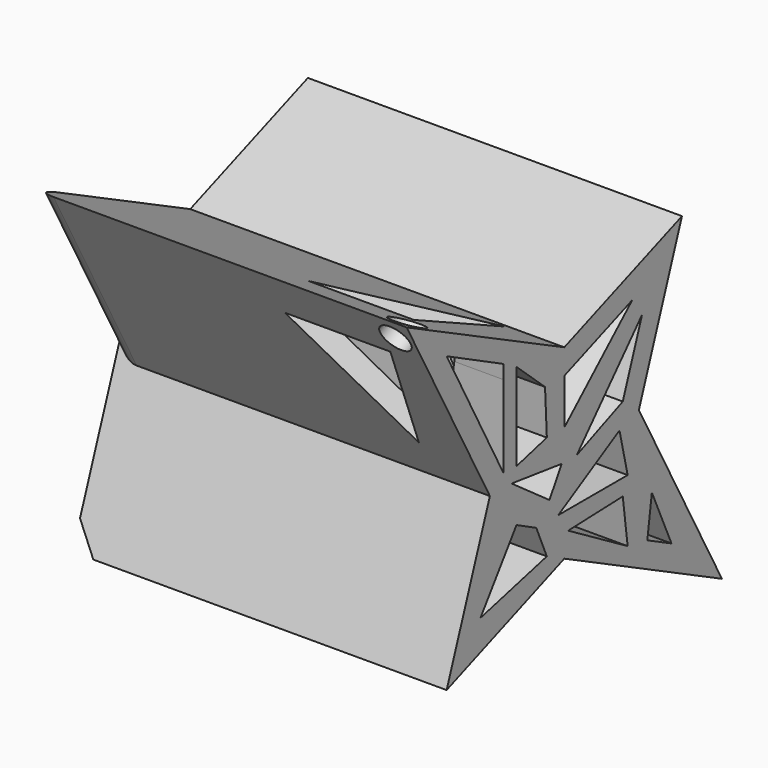
from build123d import *

# Parameters (mm, degrees)
F1_DEPTH    = 22.86
F3_DEPTH    = 22.861
F5_DEPTH    = 21.1407149532
F6_R        = 0.9322227143
F7_DEPTH    = 21.1407149532
F8_R        = 1.27
F9_T4_DEPTH = 16.1477728221


# Not quite as in the source:
# - a fillet or chamfer that OpenCascade refuses, or shapes differently, is made with other operations: its cross-section is extruded or revolved along the edge and cut away or added
# - a feature names something its author has since deleted; it is built from what else it names


with BuildPart() as f1:
    # F0 (on Right) → F1 (new body)
    with BuildSketch(Plane.YZ):
        Polygon((0, 5.6908354163), (-12.0390886441, 11.6551341489), (-5.6838279371, 0), (-8.9875673875, -9.0952031314), (0, -5.6768290866), (12.0390886441, -11.6551341489), (5.6978515349, 0), (8.9875673875, 9.0952031314), align=None)
    extrude(amount=F1_DEPTH)

    # F2 (on face) → F3 (cut, through all)
    with BuildSketch(Plane.YZ.offset(22.86)):
        Polygon((0.2947798819, -4.2920547475), (4.8379492509, -6.9700027277), (4.4653764926, -4.1452315636), align=None)
        Polygon((-0.460864554, -3.1500807424), (4.8379492509, -3.1500807424), (4.2156420195, -0.4934913878), align=None)
        Polygon((-6.4040375873, -6.2635522336), (-1.3339594007, -5.0133955665), (-2.1420896955, -3.1500807424), (-3.6510264616, -2.3839071877), align=None)
        Polygon((-3.6510264616, 0.7806772021), (-1.3339594007, 1.3762915041), (-1.4712439905, 4.1567722153), (-3.6510264616, 6.1231630373), align=None)
        Polygon((-8.9875673875, 8.8637409893), (-4.6268783625, 0.7806772021), (-4.6268783625, 5.8275670744), (-4.6572963607, 6.6916077305), align=None)
        Polygon((0.9543706066, -0.4934913878), (4.4653764926, 0.9595727897), (5.9346228684, 5.0216543911), align=None)
        Polygon((0, 1.3762915041), (5.1912929219, 6.1231630373), (0, 4.1567722153), align=None)
        Polygon((-0.1954076109, -0.4954853684), (-4.0261200629, 0), (-1.1355356546, -2.0616382826), align=None)
        Polygon((8.1868149158, -8.1874002878), (6.6878763027, -4.839763511), (6.3406112604, -7.2706225328), align=None)
    extrude(amount=-F3_DEPTH, mode=Mode.SUBTRACT)

    # F4 (on face) → F5 (cut, through all)
    with BuildSketch(Plane(origin=(0, -4.381188718, -2.3889554726), x_dir=(1, 0, 0), z_dir=(0, -0.8779615957, -0.4787310691))):
        Polygon((20.7448676229, 13.0785638466), (14.3051566556, 13.0785638466), (19.5283554494, 5.3454530425), align=None)
    extrude(amount=-F5_DEPTH, mode=Mode.SUBTRACT)

    # F6 (on face) → F7 (cut, through all)
    with BuildSketch(Plane(origin=(0, -4.381188718, -2.3889554726), x_dir=(1, 0, 0), z_dir=(0, -0.8779615957, -0.4787310691))):
        with Locations((21.6227080673, 14.5550044253)):
            Circle(F6_R)
    extrude(amount=-F7_DEPTH, mode=Mode.SUBTRACT)

    # F8
    f8_edges = [f1.edges().sort_by_distance(p)[0] for p in [
        (0, -8.861458, 5.827567),
    ]]
    fillet(f8_edges, radius=F8_R)

    # F9: chamfer of 1.27 on 1 edges, made by hand


with BuildPart() as f9_tool2:
    # F9_s3 → F9_t4 (new body)
    with BuildSketch(Plane(origin=(0, -13.9265349188, -5.2968844013), x_dir=(1, 0, 0), z_dir=(0, 0.9346765421, 0.355499313))):
        Polygon((0, 4.035998981), (1.27, 5.305998981), (0, 5.305998981), align=None)
    extrude(amount=F9_T4_DEPTH)

    split(bisect_by=Plane(origin=(0, -2.2613507756, -4.553899836), x_dir=(1, 0, 0), z_dir=(0, -0.4447575076, -0.8956510255)), keep=Keep.TOP)


with BuildPart() as f1_1:
    add(f1.part)

    # F9_t1: cut F9_tool2
    add(f9_tool2.part, mode=Mode.SUBTRACT)


solid = f1_1.part
